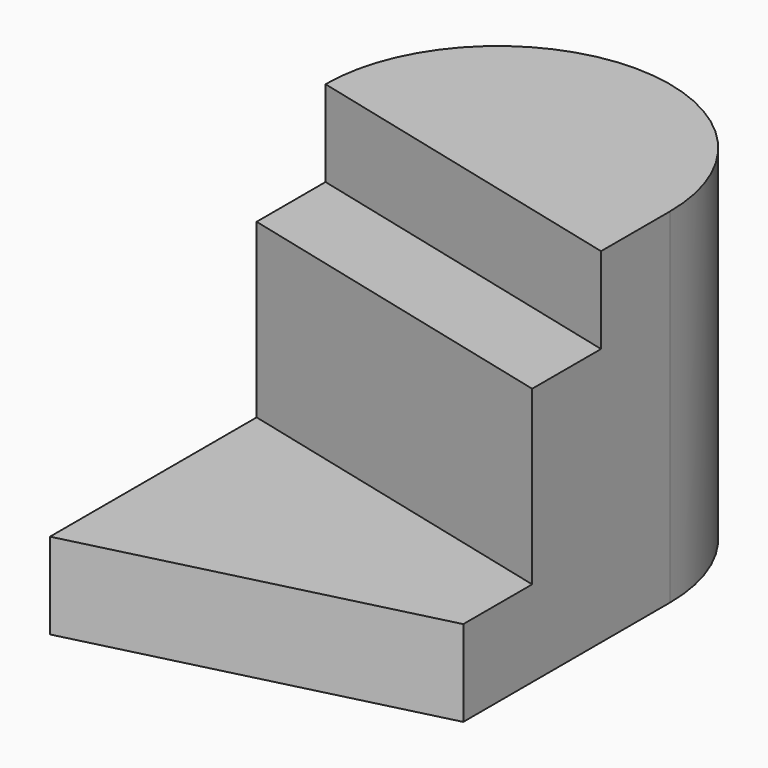
from build123d import *

# Parameters (mm, degrees)
F0_W     = 1016
F0_H     = 1016
F1_DEPTH = 1524
F3_DEPTH = 1016
F5_DEPTH = 254
F7_DEPTH = 1016
F8_DEPTH = 762


with BuildPart() as f1:
    # F0 (on Front) → F1 (new body)
    with BuildSketch(Plane.XZ):
        with Locations((-18.1896807626, 122.4249541569)):
            Rectangle(F0_W, F0_H)
    extrude(amount=F1_DEPTH)

    # F2 (on face) → F3 (cut)
    with BuildSketch(Plane.XY.offset(630.4249541569)):
        with BuildLine():
            Line((-18.1896807626, 0), (-526.1896807626, 0))
            Line((-526.1896807626, 0), (-526.1896807626, -508))
            ThreePointArc((-526.1896807626, -508), (-377.3999256054, -148.7897551572), (-18.1896807626, 0))
        make_face()
        with BuildLine():
            Line((489.8103192374, 0), (-18.1896807626, 0))
            ThreePointArc((-18.1896807626, 0), (341.0205640802, -148.7897551572), (489.8103192374, -508))
            Line((489.8103192374, -508), (489.8103192374, 0))
        make_face()
    extrude(amount=-F3_DEPTH, mode=Mode.SUBTRACT)

    # F4 (on face) → F5 (cut)
    with BuildSketch(Plane.XY.offset(630.4249541569)):
        Polygon((489.8103192374, -1016), (489.8103192374, -762), (-526.1896807626, -508), (-526.1896807626, -762), align=None)
    extrude(amount=-F5_DEPTH, mode=Mode.SUBTRACT)

    # F6 (on face) → F7 (cut)
    with BuildSketch(Plane.XY.offset(630.4249541569)):
        Polygon((489.8103192374, -1524), (489.8103192374, -1270), (-526.1896807626, -1524), align=None)
    extrude(amount=-F7_DEPTH, mode=Mode.SUBTRACT)

    # F8 (cut): a face of the model
    f8_faces = [f1.faces().sort_by_distance(p)[0] for p in [
        (-102.8563474293, -1143, 630.4249541569),
    ]]
    extrude(f8_faces, amount=-F8_DEPTH, mode=Mode.SUBTRACT)


solid = f1.part
